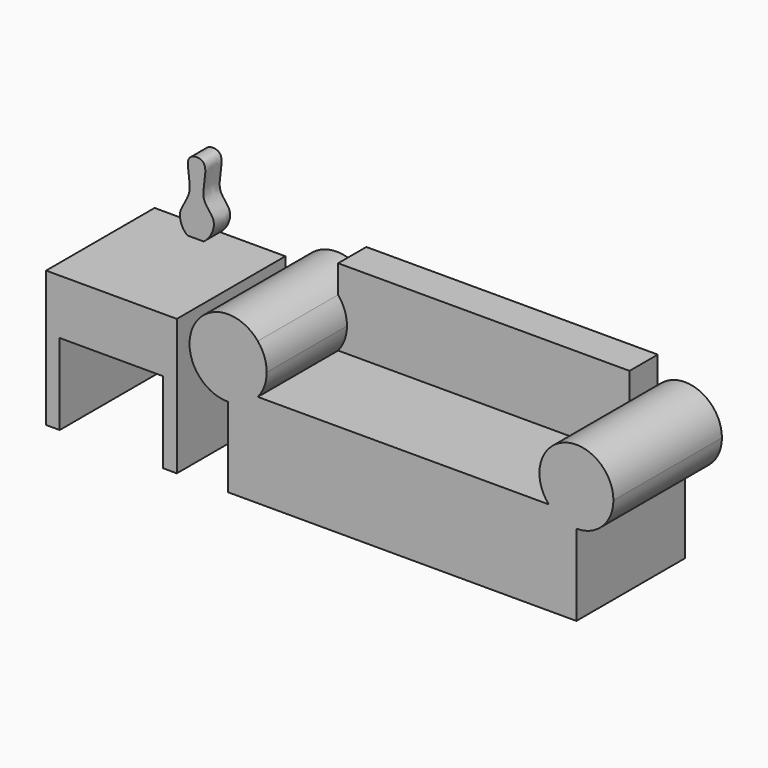
from build123d import *

# Parameters (mm, degrees)
F1_DEPTH = 25.4
F0_W     = 2.5462172925
F0_H     = 15.1793761179
F2_DEPTH = 6.604
F3_DEPTH = 3.81


with BuildPart() as f1:
    # F0 (on Front) → F1 (new body)
    with BuildSketch(Plane.XZ):
        with BuildLine():
            Line((-12.9270958542, -0.2709600874), (-12.9270958542, -15.1804022908))
            Line((-12.9270958542, -15.1804022908), (52.2952577884, -15.1804022908))
            Line((52.2952577884, -15.1804022908), (52.2952577884, 0.0293483804))
            ThreePointArc((52.2952577884, 0.0293483804), (49.4589338856, 0.636860971), (47.1202713733, 2.3528045839))
            Line((47.1202713733, 2.3528045839), (-7.3576150934, 2.3528045839))
            ThreePointArc((-7.3576150934, 2.3528045839), (-9.8488147999, 0.4178217266), (-12.9270958542, -0.2709600874))
        make_face()
        with BuildLine():
            ThreePointArc((-7.3576150934, 11.5514096105), (-19.4613812248, 10.0303881514), (-12.9270958542, -0.2709600874))
            ThreePointArc((-12.9270958542, -0.2709600874), (-9.8488147999, 0.4178217266), (-7.3576150934, 2.3528045839))
            ThreePointArc((-7.3576150934, 2.3528045839), (-6.1299849505, 4.5083430093), (-5.7040286695, 6.9521070972))
            ThreePointArc((-5.7040286695, 6.9521070972), (-6.1299849505, 9.3958711851), (-7.3576150934, 11.5514096105))
        make_face()
        with BuildLine():
            ThreePointArc((47.1202713733, 2.3528045839), (49.4589338856, 0.636860971), (52.2952577884, 0.0293483804))
            ThreePointArc((52.2952577884, 0.0293483804), (57.1918299275, 2.0575749696), (59.2200565167, 6.9541471087))
            ThreePointArc((59.2200565167, 6.9541471087), (54.8141561389, 13.4045725618), (47.2029596567, 11.6468368667))
            ThreePointArc((47.2029596567, 11.6468368667), (45.3707331109, 7.015754067), (47.1202713733, 2.3528045839))
        make_face()
    extrude(amount=F1_DEPTH)

    # F0 (on Front) → F2 (join)
    with BuildSketch(Plane.XZ):
        with BuildLine():
            Line((-7.3576150934, 16.7462788522), (-7.3576150934, 11.5514096105))
            ThreePointArc((-7.3576150934, 11.5514096105), (-6.1299849505, 9.3958711851), (-5.7040286695, 6.9521070972))
            ThreePointArc((-5.7040286695, 6.9521070972), (-6.1299849505, 4.5083430093), (-7.3576150934, 2.3528045839))
            Line((-7.3576150934, 2.3528045839), (47.1202713733, 2.3528045839))
            ThreePointArc((47.1202713733, 2.3528045839), (45.3707331109, 7.015754067), (47.2029596567, 11.6468368667))
            Line((47.2029596567, 11.6468368667), (47.2029596567, 16.7462788522))
            Line((47.2029596567, 16.7462788522), (-7.3576150934, 16.7462788522))
        make_face()
    extrude(amount=F2_DEPTH)


with BuildPart() as f1b:
    # F0 (on Front) → F1, piece 2 (new body)
    with BuildSketch(Plane.XZ):
        with BuildLine():
            Line((-37.801541388, 10.2828023955), (-47.007098794, 10.2828023955))
            Line((-47.007098794, 10.2828023955), (-47.007098794, 0))
            Line((-47.007098794, 0), (-44.4608815014, 0))
            Line((-44.4608815014, 0), (-25.0704530627, 0))
            Line((-25.0704530627, 0), (-22.5242357701, 0))
            Line((-22.5242357701, 0), (-22.5242357701, 10.2828023955))
            Line((-22.5242357701, 10.2828023955), (-34.765667282, 10.2828023955))
            add(Edge.make_bspline(
                [(-34.765667282, 10.2828023955), (-35.7584733948, 9.6059430556), (-36.9215104066, 9.6460140673), (-37.801541388, 10.2828023955)],
                knots=[0.8920605443, 0.8920605443, 0.8920605443, 0.8920605443, 1, 1, 1, 1], degree=3))
        make_face()
        with BuildLine():
            Line((-34.765667282, 10.2828023955), (-37.801541388, 10.2828023955))
            add(Edge.make_bspline(
                [(-34.765667282, 10.2828023955), (-35.7584733948, 9.6059430556), (-36.9215104066, 9.6460140673), (-37.801541388, 10.2828023955)],
                knots=[0.8920605443, 0.8920605443, 0.8920605443, 0.8920605443, 1, 1, 1, 1], degree=3))
        make_face()
        with Locations((-45.7339901477, -7.5896880589)):
            Rectangle(F0_W, F0_H)
        with Locations((-23.7973444164, -7.5896880589)):
            Rectangle(F0_W, F0_H)
    extrude(amount=F1_DEPTH)

    # F0 (on Front) → F3 (join)
    with BuildSketch(Plane.XZ):
        with BuildLine():
            add(Edge.make_bspline(
                [(-37.801541388, 10.2828023955), (-38.7599736077, 10.9763216736), (-40.0908364875, 13.9709710064), (-36.2154597414, 17.4726187492), (-38.9577883228, 23.8943574963), (-33.1299998967, 24.0180152523), (-36.0866597264, 16.9616831482), (-31.7508708707, 14.6440412886), (-33.5790707592, 11.0917810359), (-34.765667282, 10.2828023955)],
                knots=[0, 0, 0, 0, 0.1175556933, 0.2512234277, 0.3936845222, 0.4944197281, 0.6420629054, 0.7630518878, 0.8920605443, 0.8920605443, 0.8920605443, 0.8920605443], degree=3))
            Line((-37.801541388, 10.2828023955), (-34.765667282, 10.2828023955))
        make_face()
        with BuildLine():
            Line((-34.765667282, 10.2828023955), (-37.801541388, 10.2828023955))
            add(Edge.make_bspline(
                [(-34.765667282, 10.2828023955), (-35.7584733948, 9.6059430556), (-36.9215104066, 9.6460140673), (-37.801541388, 10.2828023955)],
                knots=[0.8920605443, 0.8920605443, 0.8920605443, 0.8920605443, 1, 1, 1, 1], degree=3))
        make_face()
    extrude(amount=F3_DEPTH)


solid = Compound([f1.part, f1b.part])
